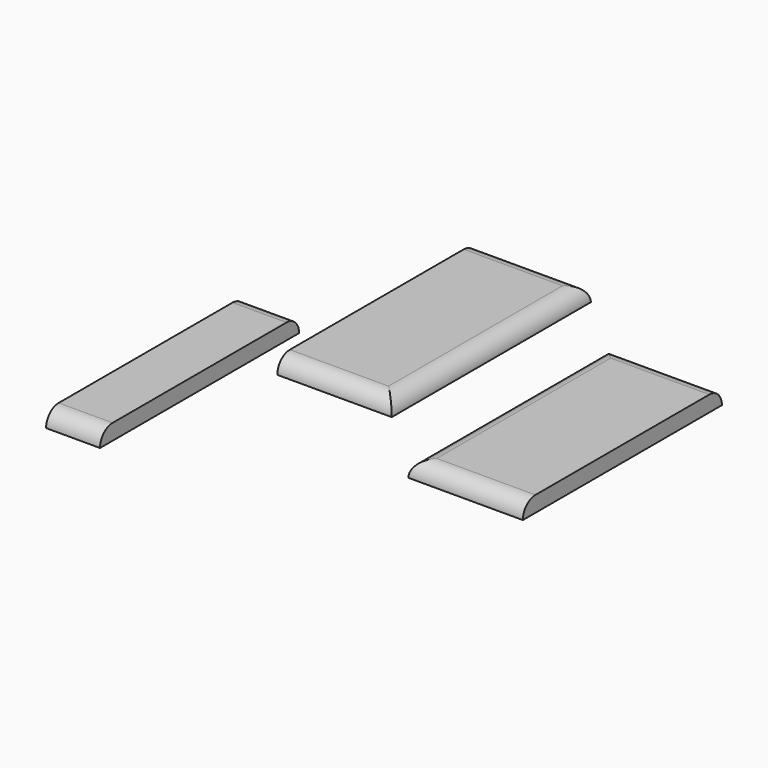
from build123d import *

# Parameters (mm, degrees)
F0_W     = 138
F0_H     = 300
F1_DEPTH = 19
F2_W     = 65
F2_H     = 300
F3_DEPTH = 19
F4_W     = 138
F4_H     = 300
F5_DEPTH = 19
F6_R     = 18.99999
F6_2_R   = 18.99999
F6_3_R   = 18.99999


# Not quite as in the source:
# - a fillet or chamfer is up to 0.001 mm smaller than in the source, because OpenCascade refuses the exact size


with BuildPart() as f1:
    # F0 (on Top) → F1 (new body)
    with BuildSketch(Plane.XY):
        with Locations((-77.230250597, 70.7261949778)):
            Rectangle(F0_W, F0_H)
    extrude(amount=F1_DEPTH)

    # F6#2 (radius 19 in the source; OpenCascade refuses exactly that, so slightly less here)
    f6_2_edges = [f1.edges().sort_by_distance(p)[0] for p in [
        (-77.230251, -79.273805, 19),
        (-8.230251, 70.726195, 19),
        (-77.230251, 220.726195, 19),
    ]]
    fillet(f6_2_edges, radius=F6_2_R)


with BuildPart() as f3:
    # F2 (on Top) → F3 (new body)
    with BuildSketch(Plane.XY):
        with Locations((-215.8502775431, -150)):
            Rectangle(F2_W, F2_H)
    extrude(amount=F3_DEPTH)

    # F6 (radius 19 in the source; OpenCascade refuses exactly that, so slightly less here)
    f6_edges = [f3.edges().sort_by_distance(p)[0] for p in [
        (-215.850278, 0, 19),
        (-215.850278, -300, 19),
    ]]
    fillet(f6_edges, radius=F6_R)


with BuildPart() as f5:
    # F4 (on Top) → F5 (new body)
    with BuildSketch(Plane.XY):
        with Locations((150.2515169382, -16.0771518946)):
            Rectangle(F4_W, F4_H)
    extrude(amount=F5_DEPTH)

    # F6#3 (radius 19 in the source; OpenCascade refuses exactly that, so slightly less here)
    f6_3_edges = [f5.edges().sort_by_distance(p)[0] for p in [
        (150.251517, 133.922848, 19),
        (81.251517, -16.077152, 19),
        (150.251517, -166.077152, 19),
    ]]
    fillet(f6_3_edges, radius=F6_3_R)


solid = Compound([f1.part, f3.part, f5.part])
